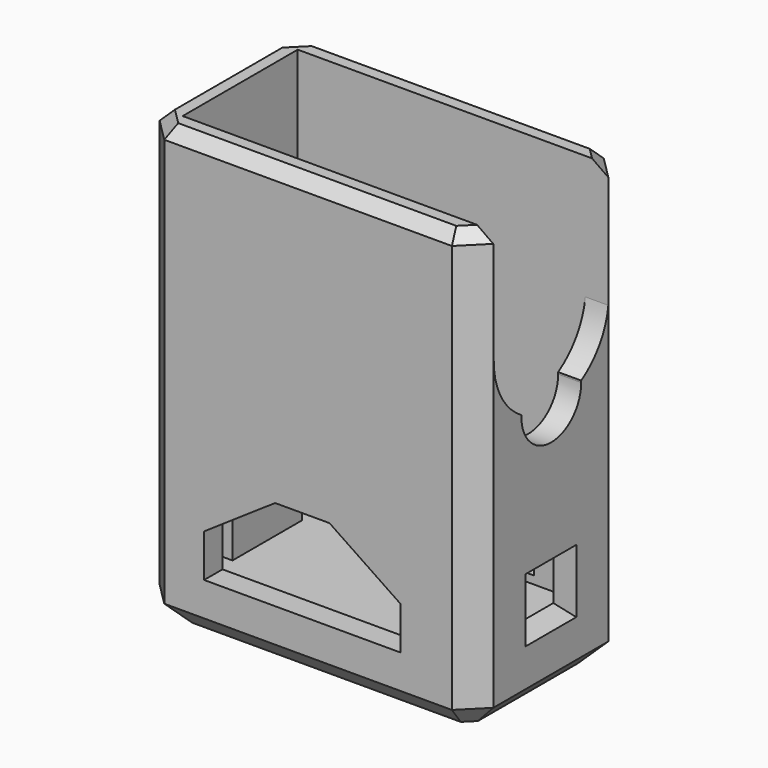
from build123d import *

# Parameters (mm, degrees)
F0_W      = 29
F0_H      = 16.5
F1_DEPTH  = 38.5
F2_SIZE   = 2
F3_SIZE   = 2
F4_SIZE   = 1
F5_W      = 25
F5_H      = 12.5
F6_DEPTH  = 34.25
F8_DEPTH  = 16.501
F9_W      = 12.5
F9_H      = 1
F10_DEPTH = 25
F11_W     = 7.54
F11_H     = 7.25
F11_R     = 1.1
F12_DEPTH = 4.35
F13_R     = 2
F14_DEPTH = 25
F15_W     = 5.538
F15_H     = 5.533
F17_W     = 5.538
F17_H     = 4.538


with BuildPart() as f1:
    # F0 (on Top) → F1 (new body)
    with BuildSketch(Plane.XY):
        with Locations((14.5, 8.25)):
            Rectangle(F0_W, F0_H)
    extrude(amount=F1_DEPTH)

    # F2
    f2_edges = [f1.edges().sort_by_distance(p)[0] for p in [
        (0, 0, 19.25),
        (0, 16.5, 19.25),
        (29, 0, 19.25),
        (29, 16.5, 19.25),
    ]]
    chamfer(f2_edges, length=F2_SIZE)

    # F3
    f3_edges = [f1.edges().sort_by_distance(p)[0] for p in [
        (0, 8.25, 0),
        (1, 15.5, 0),
        (1, 1, 0),
        (14.5, 16.5, 0),
        (14.5, 0, 0),
        (28, 15.5, 0),
        (28, 1, 0),
        (29, 8.25, 0),
    ]]
    chamfer(f3_edges, length=F3_SIZE)

    # F4
    f4_edges = [f1.edges().sort_by_distance(p)[0] for p in [
        (0, 8.25, 38.5),
        (1, 15.5, 38.5),
        (1, 1, 38.5),
        (14.5, 16.5, 38.5),
        (14.5, 0, 38.5),
        (28, 15.5, 38.5),
        (28, 1, 38.5),
        (29, 8.25, 38.5),
    ]]
    chamfer(f4_edges, length=F4_SIZE)

    # F5 (on face) → F6 (cut)
    with BuildSketch(Plane.XY.offset(38.5)):
        with Locations((14.5, 8.25)):
            Rectangle(F5_W, F5_H)
    extrude(amount=-F6_DEPTH, mode=Mode.SUBTRACT)

    # F7 (on face) → F8 (cut, through all)
    with BuildSketch(Plane.XZ):
        Polygon((5.464, 8.664), (5.464, 4.94), (22.536, 4.94), (22.536, 8.664), (16.364, 12.836), (11.636, 12.836), align=None)
    extrude(amount=-F8_DEPTH, mode=Mode.SUBTRACT)

    # F9 (on face) → F10 (cut)
    with BuildSketch(Plane.YZ.offset(29)):
        with BuildLine():
            ThreePointArc((5.0538961688, 23.1590909091), (8.2204306945, 19.7509741882), (11.55, 23))
            ThreePointArc((11.55, 23), (11.5490258118, 23.0795693055), (11.5461038312, 23.1590909091))
            ThreePointArc((11.5461038312, 23.1590909091), (8.3, 22.25), (5.0538961688, 23.1590909091))
        make_face()
        with BuildLine():
            ThreePointArc((5.0538961688, 23.1590909091), (8.3, 22.25), (11.5461038312, 23.1590909091))
            ThreePointArc((11.5461038312, 23.1590909091), (8.3, 26.25), (5.0538961688, 23.1590909091))
        make_face()
        with BuildLine():
            ThreePointArc((5.0538961688, 23.1590909091), (8.3, 26.25), (11.5461038312, 23.1590909091))
            ThreePointArc((11.5461038312, 23.1590909091), (13.5428254576, 25.0977535038), (14.5, 27.7110133081))
            Line((14.5, 27.7110133081), (14.5, 28.5))
            Line((14.5, 28.5), (2.05, 28.5))
            ThreePointArc((2.05, 28.5), (2.8524937382, 25.4361502113), (5.0538961688, 23.1590909091))
        make_face()
        with BuildLine():
            Line((2, 28.5), (2.05, 28.5))
            ThreePointArc((2.05, 28.5), (7.9047152925, 34.7374874749), (14.5, 29.2889866919))
            Line((14.5, 29.2889866919), (14.5, 37.5))
            Line((14.5, 37.5), (2, 37.5))
            Line((2, 37.5), (2, 28.5))
        make_face()
        with BuildLine():
            ThreePointArc((14.5, 29.2889866919), (7.9047152925, 34.7374874749), (2.05, 28.5))
            Line((2.05, 28.5), (14.5, 28.5))
            Line((14.5, 28.5), (14.5, 29.2889866919))
        make_face()
        with Locations((8.25, 38)):
            Rectangle(F9_W, F9_H)
    extrude(amount=-F10_DEPTH, mode=Mode.SUBTRACT)

    # F11 (on face) → F12 (join)
    with BuildSketch(Plane(origin=(0, 0, 0), x_dir=(0, -1, 0), z_dir=(-1, 0, 0))):
        with Locations((-8.25, 7.875)):
            Rectangle(F11_W, F11_H)
        with Locations((-8.25, 9)):
            Circle(F11_R, mode=Mode.SUBTRACT)
    extrude(amount=-F12_DEPTH)

    # F13 (on face) → F14 (cut)
    with BuildSketch(Plane.YZ.offset(2)):
        with Locations((8.25, 22.9216944426)):
            Circle(F13_R)
    extrude(amount=-F14_DEPTH, mode=Mode.SUBTRACT)

    # F15 (on face) → F18 section 0
    with BuildSketch(Plane.YZ.offset(29)):
        with Locations((8.25, 8.0385)):
            Rectangle(F15_W, F15_H)
    # F17 (on offset) → F18 section 1
    with BuildSketch(Plane.YZ.offset(24.55)):
        with Locations((8.25, 8.491)):
            Rectangle(F17_W, F17_H)
    loft(mode=Mode.SUBTRACT)


solid = f1.part
